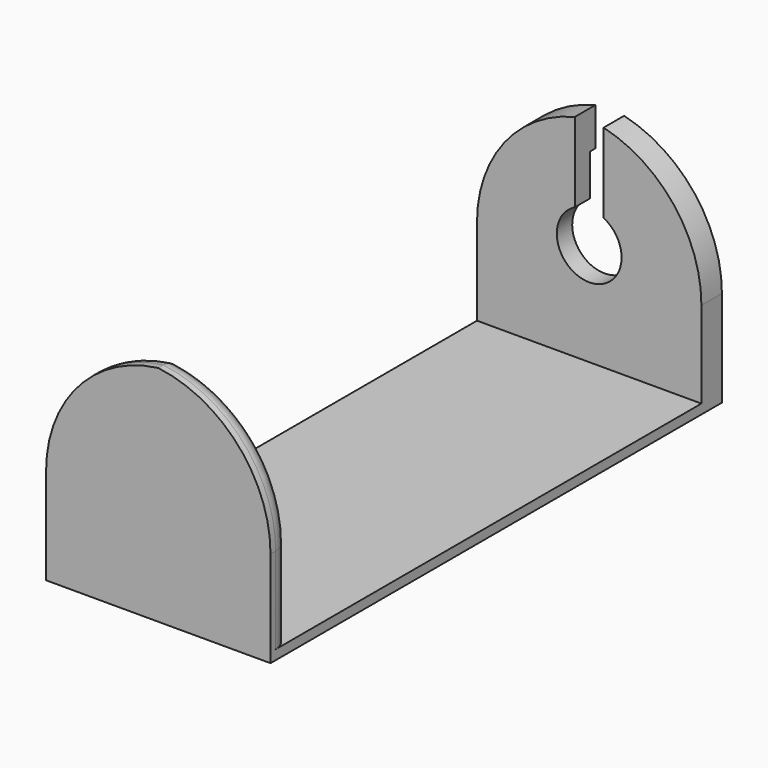
from build123d import *

# Parameters (mm, degrees)
F1_DEPTH    = 17.5
F2_T1_DEPTH = 104
F2_T3_DEPTH = 104
F4_DEPTH    = 1
F5_DEPTH    = 25
F6_R        = 3


# Not quite as in the source:
# - a fillet or chamfer that OpenCascade refuses, or shapes differently, is made with other operations: its cross-section is extruded or revolved along the edge and cut away or added


with BuildPart() as f1:
    # F0 (on Right) → F1 (new body, symmetric)
    with BuildSketch(Plane.YZ):
        Polygon((-44, 35), (-44, 0), (44, 0), (44, 35), (40, 35), (40, 1.5), (-40, 1.5), (-40, 35), align=None)
    extrude(amount=F1_DEPTH, both=True)

    # F2: fillet of radius 20 on 4 edges, made by hand

    # F2_s2 → F2_t1 (cut)
    with BuildSketch(Plane.XZ.offset(-94)):
        with BuildLine():
            ThreePointArc((-2.5, 35), (11.6421356237, 29.1421356237), (17.5, 15))
            Line((17.5, 15), (17.5, 35))
            Line((17.5, 35), (-2.5, 35))
        make_face()
        with BuildLine():
            ThreePointArc((2.5, 35), (-11.6421356237, 29.1421356237), (-17.5, 15))
            Line((-17.5, 15), (-17.5, 35))
            Line((-17.5, 35), (2.5, 35))
        make_face()
    extrude(amount=F2_T1_DEPTH, mode=Mode.SUBTRACT)

    # F2_s4 → F2_t3 (cut)
    with BuildSketch(Plane.XZ.offset(-10)):
        with BuildLine():
            ThreePointArc((2.5, 35), (-11.6421356237, 29.1421356237), (-17.5, 15))
            Line((-17.5, 15), (-17.5, 35))
            Line((-17.5, 35), (2.5, 35))
        make_face()
        with BuildLine():
            ThreePointArc((-2.5, 35), (11.6421356237, 29.1421356237), (17.5, 15))
            Line((17.5, 15), (17.5, 35))
            Line((17.5, 35), (-2.5, 35))
        make_face()
    extrude(amount=F2_T3_DEPTH, mode=Mode.SUBTRACT)

    # F3 (on face) → F4 (cut)
    with BuildSketch(Plane(origin=(0, 44, 0), x_dir=(-1, 0, 0), z_dir=(0, 1, 0))):
        with BuildLine():
            Line((2.25, 22.0293655688), (2.25, 28.4799718057))
            ThreePointArc((2.25, 28.4799718057), (0, 28.7083037466), (-2.25, 28.4799718057))
            Line((-2.25, 28.4799718057), (-2.25, 22.0293655688))
            ThreePointArc((-2.25, 22.0293655688), (0, 12.4583037466), (2.25, 22.0293655688))
        make_face()
        with BuildLine():
            ThreePointArc((-2.25, 28.4799718057), (-7.0795480082, 8.8295941651), (11.2, 17.5083037466))
            ThreePointArc((11.2, 17.5083037466), (8.6787095815, 24.5878517548), (2.25, 28.4799718057))
            Line((2.25, 28.4799718057), (2.25, 22.0293655688))
            ThreePointArc((2.25, 22.0293655688), (0, 12.4583037466), (-2.25, 22.0293655688))
            Line((-2.25, 22.0293655688), (-2.25, 28.4799718057))
        make_face()
    extrude(amount=-F4_DEPTH, mode=Mode.SUBTRACT)

    # F3 (on face) → F5 (cut)
    with BuildSketch(Plane(origin=(0, 44, 0), x_dir=(-1, 0, 0), z_dir=(0, 1, 0))):
        with BuildLine():
            Line((2.25, 22.0293655688), (2.25, 28.4799718057))
            ThreePointArc((2.25, 28.4799718057), (0, 28.7083037466), (-2.25, 28.4799718057))
            Line((-2.25, 28.4799718057), (-2.25, 22.0293655688))
            ThreePointArc((-2.25, 22.0293655688), (0, 12.4583037466), (2.25, 22.0293655688))
        make_face()
        with BuildLine():
            ThreePointArc((-2.25, 28.4799718057), (0, 28.7083037466), (2.25, 28.4799718057))
            Line((2.25, 28.4799718057), (2.25, 34.4277507705))
            ThreePointArc((2.25, 34.4277507705), (1.1309449156, 34.6676444705), (0, 34.843134833))
            ThreePointArc((0, 34.843134833), (-1.1309449156, 34.6676444705), (-2.25, 34.4277507705))
            Line((-2.25, 34.4277507705), (-2.25, 28.4799718057))
        make_face()
    extrude(amount=-F5_DEPTH, mode=Mode.SUBTRACT)

    # F6
    f6_edges = [f1.edges().sort_by_distance(p)[0] for p in [
        (17.5, -40, 8.25),
        (-17.5, -40, 8.25),
    ]]
    fillet(f6_edges, radius=F6_R)


solid = f1.part
